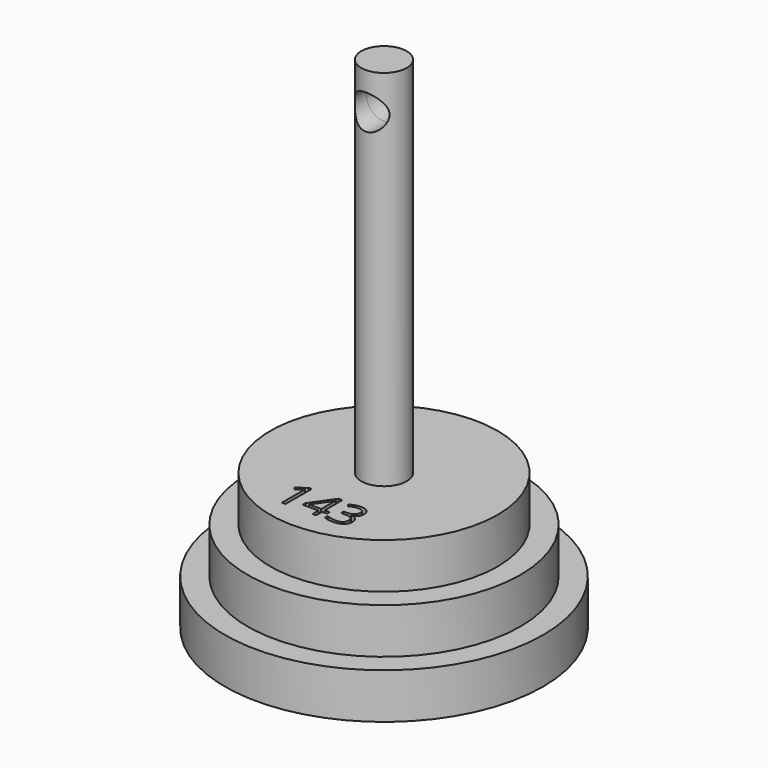
from build123d import *

# Parameters (mm, degrees)
F0_R          = 22.225
F1_DEPTH      = 6.35
F2_R          = 19.05
F3_DEPTH      = 6.35
F4_R          = 15.875
F5_DEPTH      = 6.35
F6_R          = 3.175
F7_DEPTH      = 50.8
F8_R          = 2.4196550367
F9_DEPTH      = 25.4
F9_DEPTH_BACK = 25.4
F10_TEXT_SIZE = 6.3840946597
F11_DEPTH     = 6.35
F12_TEXT_SIZE = 5.3770154611
F13_DEPTH     = 6.35


# Not quite as in the source:
# - Text() gives the source's letters only with a copy of the font that has no kerning and outlines rounded to 1/6400 em; it was checked with that copy


with BuildPart() as f1:
    # F0 (on Top) → F1 (new body)
    with BuildSketch(Plane.XY):
        Circle(F0_R)
    extrude(amount=F1_DEPTH)

    # F2 (on face) → F3 (join)
    with BuildSketch(Plane.XY.offset(6.35)):
        Circle(F2_R)
    extrude(amount=F3_DEPTH)

    # F4 (on face) → F5 (join)
    with BuildSketch(Plane.XY.offset(12.7)):
        Circle(F4_R)
    extrude(amount=F5_DEPTH)

    # F6 (on face) → F7 (join)
    with BuildSketch(Plane.XY.offset(19.05)):
        Circle(F6_R)
    extrude(amount=F7_DEPTH)

    # F8 (on Front) → F9 (cut, two sides)
    with BuildSketch(Plane.XZ) as f9_sk:
        with Locations((0, 64.6855041268)):
            Circle(F8_R)
    extrude(amount=-F9_DEPTH, mode=Mode.SUBTRACT)
    extrude(f9_sk.sketch, amount=F9_DEPTH_BACK, mode=Mode.SUBTRACT)

    # F10 (on face) → F11 (cut)
    with BuildSketch(Plane.XY.offset(19.05)):
        with Locations((-6.0111279599, -12.4562019482)):
            Text('143', F10_TEXT_SIZE, font='Open Sans', text_align=(TextAlign.LEFT, TextAlign.BOTTOM))
    extrude(amount=-F11_DEPTH, mode=Mode.SUBTRACT)

    # F12 (on face) → F13 (cut)
    with BuildSketch(Plane(origin=(0, 0, 0), x_dir=(1, 0, 0), z_dir=(0, 0, -1))):
        with Locations((-2.8390642256, -18.3248696849)):
            Text('-b', F12_TEXT_SIZE, font='Open Sans', text_align=(TextAlign.LEFT, TextAlign.BOTTOM))
    extrude(amount=-F13_DEPTH, mode=Mode.SUBTRACT)


solid = f1.part
